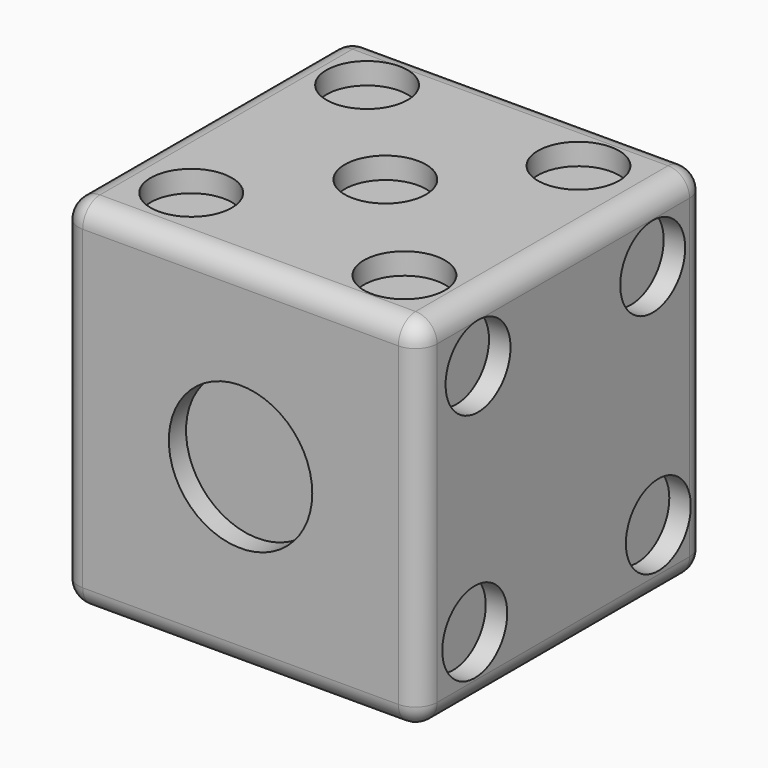
from build123d import *

# Parameters (mm, degrees)
F0_W          = 12.7
F0_H          = 12.7
F1_DEPTH      = 12.7
F2_R          = 2.54
F3_DEPTH      = 0.762
F4_R          = 1.4370558
F5_DEPTH      = 0.762
F6_R          = 1.4370558
F7_DEPTH      = 0.762
F8_R          = 1.4370558
F9_DEPTH      = 0.762
F10_R         = 1.4370558
F11_DEPTH     = 0.762
F12_T1_DEPTH  = 11.176
F12_T3_DEPTH  = 11.176
F12_T5_DEPTH  = 11.176
F12_S9_W      = 0.762
F12_S9_H      = 0.762
F12_T10_DEPTH = 0.762
F12_S15_W     = 0.762
F12_S15_H     = 0.762
F12_T16_DEPTH = 0.762
F12_S21_W     = 0.762
F12_S21_H     = 0.762
F12_T22_DEPTH = 0.762
F12_S27_W     = 0.762
F12_S27_H     = 0.762
F12_T28_DEPTH = 0.762
F12_S33_W     = 0.762
F12_S33_H     = 0.762
F12_T34_DEPTH = 0.762
F12_S39_W     = 0.762
F12_S39_H     = 0.762
F12_T40_DEPTH = 0.762
F12_S45_W     = 0.762
F12_S45_H     = 0.762
F12_T46_DEPTH = 0.762
F12_S51_W     = 0.762
F12_S51_H     = 0.762
F12_T52_DEPTH = 0.762
F13_R         = 1.4370558
F14_DEPTH     = 0.762


# Not quite as in the source:
# - a fillet or chamfer that OpenCascade refuses, or shapes differently, is made with other operations: its cross-section is extruded or revolved along the edge and cut away or added


with BuildPart() as f1:
    # F0 (on Front) → F1 (new body)
    with BuildSketch(Plane.XZ):
        Rectangle(F0_W, F0_H)
    extrude(amount=F1_DEPTH)

    # F2 (on face) → F3 (cut)
    with BuildSketch(Plane.XZ.offset(12.7)):
        Circle(F2_R)
    extrude(amount=-F3_DEPTH, mode=Mode.SUBTRACT)

    # F4 (on face) → F5 (cut)
    with BuildSketch(Plane(origin=(0, 0, 0), x_dir=(-1, 0, 0), z_dir=(0, 1, 0))):
        with Locations((-4.0605822578, 4.3273498304)):
            Circle(F4_R)
        with Locations((4.0411474183, -3.9733615704)):
            Circle(F4_R)
    extrude(amount=-F5_DEPTH, mode=Mode.SUBTRACT)

    # F6 (on face) → F7 (cut)
    with BuildSketch(Plane(origin=(-6.35, 0, 0), x_dir=(0, -1, 0), z_dir=(-1, 0, 0))):
        with Locations((6.2880520709, 0)):
            Circle(F6_R)
        with Locations((10.5908196419, -4.2169503868)):
            Circle(F6_R)
        with Locations((2.0048597362, 4.2917155661)):
            Circle(F6_R)
    extrude(amount=-F7_DEPTH, mode=Mode.SUBTRACT)

    # F8 (on face) → F9 (cut)
    with BuildSketch(Plane.YZ.offset(6.35)):
        with Locations((-10.1248482242, 4.1586253792)):
            Circle(F8_R)
        with Locations((-2.3929197341, 4.1189542972)):
            Circle(F8_R)
        with Locations((-10.2693093941, -4.0696617216)):
            Circle(F8_R)
        with Locations((-2.1438063122, -4.0340232663)):
            Circle(F8_R)
    extrude(amount=-F9_DEPTH, mode=Mode.SUBTRACT)

    # F10 (on face) → F11 (cut)
    with BuildSketch(Plane.XY.offset(6.35)):
        with Locations((0, -6.2898481265)):
            Circle(F10_R)
        with Locations((3.6543684546, -2.3101689294)):
            Circle(F10_R)
        with Locations((-3.9310273714, -2.1862694994)):
            Circle(F10_R)
        with Locations((-3.6943627056, -10.2638797835)):
            Circle(F10_R)
        with Locations((3.9920811541, -10.4369977489)):
            Circle(F10_R)
    extrude(amount=-F11_DEPTH, mode=Mode.SUBTRACT)

    # F12: fillet of radius 0.762 on 12 edges, made by hand

    # F12_s2 → F12_t1 (cut)
    with BuildSketch(Plane.YZ.offset(-5.588)):
        with BuildLine():
            ThreePointArc((-11.938, 6.35), (-12.4768153673, 6.1268153673), (-12.7, 5.588))
            Line((-12.7, 5.588), (-12.7, 6.35))
            Line((-12.7, 6.35), (-11.938, 6.35))
        make_face()
        with BuildLine():
            ThreePointArc((-0.762, 6.35), (-0.2231846327, 6.1268153673), (0, 5.588))
            Line((0, 5.588), (0, 6.35))
            Line((0, 6.35), (-0.762, 6.35))
        make_face()
        with BuildLine():
            ThreePointArc((-12.7, -5.588), (-12.4768153673, -6.1268153673), (-11.938, -6.35))
            Line((-11.938, -6.35), (-12.7, -6.35))
            Line((-12.7, -6.35), (-12.7, -5.588))
        make_face()
        with BuildLine():
            ThreePointArc((0, -5.588), (-0.2231846327, -6.1268153673), (-0.762, -6.35))
            Line((-0.762, -6.35), (0, -6.35))
            Line((0, -6.35), (0, -5.588))
        make_face()
    extrude(amount=F12_T1_DEPTH, mode=Mode.SUBTRACT)

    # F12_s4 → F12_t3 (cut)
    with BuildSketch(Plane.XZ.offset(0.762)):
        with BuildLine():
            ThreePointArc((-5.588, 6.35), (-6.1268153673, 6.1268153673), (-6.35, 5.588))
            Line((-6.35, 5.588), (-6.35, 6.35))
            Line((-6.35, 6.35), (-5.588, 6.35))
        make_face()
        with BuildLine():
            ThreePointArc((5.588, 6.35), (6.1268153673, 6.1268153673), (6.35, 5.588))
            Line((6.35, 5.588), (6.35, 6.35))
            Line((6.35, 6.35), (5.588, 6.35))
        make_face()
        with BuildLine():
            ThreePointArc((6.35, -5.588), (6.1268153673, -6.1268153673), (5.588, -6.35))
            Line((5.588, -6.35), (6.35, -6.35))
            Line((6.35, -6.35), (6.35, -5.588))
        make_face()
        with BuildLine():
            ThreePointArc((-6.35, -5.588), (-6.1268153673, -6.1268153673), (-5.588, -6.35))
            Line((-5.588, -6.35), (-6.35, -6.35))
            Line((-6.35, -6.35), (-6.35, -5.588))
        make_face()
    extrude(amount=F12_T3_DEPTH, mode=Mode.SUBTRACT)

    # F12_s6 → F12_t5 (cut)
    with BuildSketch(Plane.XY.offset(-5.588)):
        with BuildLine():
            ThreePointArc((6.35, -11.938), (6.1268153673, -12.4768153673), (5.588, -12.7))
            Line((5.588, -12.7), (6.35, -12.7))
            Line((6.35, -12.7), (6.35, -11.938))
        make_face()
        with BuildLine():
            ThreePointArc((-5.588, -12.7), (-6.1268153673, -12.4768153673), (-6.35, -11.938))
            Line((-6.35, -11.938), (-6.35, -12.7))
            Line((-6.35, -12.7), (-5.588, -12.7))
        make_face()
        with BuildLine():
            ThreePointArc((6.35, -0.762), (6.1268153673, -0.2231846327), (5.588, 0))
            Line((5.588, 0), (6.35, 0))
            Line((6.35, 0), (6.35, -0.762))
        make_face()
        with BuildLine():
            ThreePointArc((-5.588, 0), (-6.1268153673, -0.2231846327), (-6.35, -0.762))
            Line((-6.35, -0.762), (-6.35, 0))
            Line((-6.35, 0), (-5.588, 0))
        make_face()
    extrude(amount=F12_T5_DEPTH, mode=Mode.SUBTRACT)


with BuildPart() as f12_tool8:
    # F12_s9 → F12_t10 (new body)
    with BuildSketch(Plane.XY.offset(5.588)):
        with Locations((5.969, -12.319)):
            Rectangle(F12_S9_W, F12_S9_H)
    extrude(amount=F12_T10_DEPTH)

    # F12_s11 → F12_t12 (revolve, cut)
    with BuildSketch(Plane(origin=(5.588, -11.938, 5.588), x_dir=(-0.7071067812, 0.7071067812, 0), z_dir=(0.7071067812, 0.7071067812, 0))):
        with BuildLine():
            ThreePointArc((0, -0.762), (0.762, 0), (0, 0.762))
            Line((0, 0.762), (0, -0.762))
        make_face()
    revolve(axis=Axis((5.588, -11.938, 5.588), (0, 0, 1)), mode=Mode.SUBTRACT)


with BuildPart() as f1_1:
    add(f1.part)

    # F12_t7: cut F12_tool8
    add(f12_tool8.part, mode=Mode.SUBTRACT)


with BuildPart() as f12_tool14:
    # F12_s15 → F12_t16 (new body)
    with BuildSketch(Plane.XY.offset(5.588)):
        with Locations((-5.969, -12.319)):
            Rectangle(F12_S15_W, F12_S15_H)
    extrude(amount=F12_T16_DEPTH)

    # F12_s17 → F12_t18 (revolve, cut)
    with BuildSketch(Plane(origin=(-5.588, -11.938, 5.588), x_dir=(0.7071067812, 0.7071067812, 0), z_dir=(0.7071067812, -0.7071067812, 0))):
        with BuildLine():
            ThreePointArc((0, -0.762), (0.762, 0), (0, 0.762))
            Line((0, 0.762), (0, -0.762))
        make_face()
    revolve(axis=Axis((-5.588, -11.938, 5.588), (0, 0, 1)), mode=Mode.SUBTRACT)


with BuildPart() as f1_2:
    add(f1_1.part)

    # F12_t13: cut F12_tool14
    add(f12_tool14.part, mode=Mode.SUBTRACT)


with BuildPart() as f12_tool20:
    # F12_s21 → F12_t22 (new body)
    with BuildSketch(Plane.XY.offset(5.588)):
        with Locations((-5.969, -0.381)):
            Rectangle(F12_S21_W, F12_S21_H)
    extrude(amount=F12_T22_DEPTH)

    # F12_s23 → F12_t24 (revolve, cut)
    with BuildSketch(Plane(origin=(-5.588, -0.762, 5.588), x_dir=(0.7071067812, -0.7071067812, 0), z_dir=(-0.7071067812, -0.7071067812, 0))):
        with BuildLine():
            ThreePointArc((0, -0.762), (0.762, 0), (0, 0.762))
            Line((0, 0.762), (0, -0.762))
        make_face()
    revolve(axis=Axis((-5.588, -0.762, 5.588), (0, 0, 1)), mode=Mode.SUBTRACT)


with BuildPart() as f1_3:
    add(f1_2.part)

    # F12_t19: cut F12_tool20
    add(f12_tool20.part, mode=Mode.SUBTRACT)


with BuildPart() as f12_tool26:
    # F12_s27 → F12_t28 (new body)
    with BuildSketch(Plane.XY.offset(5.588)):
        with Locations((5.969, -0.381)):
            Rectangle(F12_S27_W, F12_S27_H)
    extrude(amount=F12_T28_DEPTH)

    # F12_s29 → F12_t30 (revolve, cut)
    with BuildSketch(Plane(origin=(5.588, -0.762, 5.588), x_dir=(-0.7071067812, -0.7071067812, 0), z_dir=(-0.7071067812, 0.7071067812, 0))):
        with BuildLine():
            ThreePointArc((0, -0.762), (0.762, 0), (0, 0.762))
            Line((0, 0.762), (0, -0.762))
        make_face()
    revolve(axis=Axis((5.588, -0.762, 5.588), (0, 0, 1)), mode=Mode.SUBTRACT)


with BuildPart() as f1_4:
    add(f1_3.part)

    # F12_t25: cut F12_tool26
    add(f12_tool26.part, mode=Mode.SUBTRACT)


with BuildPart() as f12_tool32:
    # F12_s33 → F12_t34 (new body)
    with BuildSketch(Plane.YZ.offset(5.588)):
        with Locations((-12.319, -5.969)):
            Rectangle(F12_S33_W, F12_S33_H)
    extrude(amount=F12_T34_DEPTH)

    # F12_s35 → F12_t36 (revolve, cut)
    with BuildSketch(Plane(origin=(5.588, -11.938, -5.588), x_dir=(0, 0.7071067812, 0.7071067812), z_dir=(0, 0.7071067812, -0.7071067812))):
        with BuildLine():
            ThreePointArc((0, -0.762), (0.762, 0), (0, 0.762))
            Line((0, 0.762), (0, -0.762))
        make_face()
    revolve(axis=Axis((5.588, -11.938, -5.588), (1, 0, 0)), mode=Mode.SUBTRACT)


with BuildPart() as f1_5:
    add(f1_4.part)

    # F12_t31: cut F12_tool32
    add(f12_tool32.part, mode=Mode.SUBTRACT)


with BuildPart() as f12_tool38:
    # F12_s39 → F12_t40 (new body)
    with BuildSketch(Plane.XY.offset(-5.588)):
        with Locations((-5.969, -12.319)):
            Rectangle(F12_S39_W, F12_S39_H)
    extrude(amount=-F12_T40_DEPTH)

    # F12_s41 → F12_t42 (revolve, cut)
    with BuildSketch(Plane(origin=(-5.588, -11.938, -5.588), x_dir=(0.7071067812, 0.7071067812, 0), z_dir=(-0.7071067812, 0.7071067812, 0))):
        with BuildLine():
            ThreePointArc((0, -0.762), (0.762, 0), (0, 0.762))
            Line((0, 0.762), (0, -0.762))
        make_face()
    revolve(axis=Axis((-5.588, -11.938, -5.588), (0, 0, -1)), mode=Mode.SUBTRACT)


with BuildPart() as f1_6:
    add(f1_5.part)

    # F12_t37: cut F12_tool38
    add(f12_tool38.part, mode=Mode.SUBTRACT)


with BuildPart() as f12_tool44:
    # F12_s45 → F12_t46 (new body)
    with BuildSketch(Plane.YZ.offset(5.588)):
        with Locations((-0.381, -5.969)):
            Rectangle(F12_S45_W, F12_S45_H)
    extrude(amount=F12_T46_DEPTH)

    # F12_s47 → F12_t48 (revolve, cut)
    with BuildSketch(Plane(origin=(5.588, -0.762, -5.588), x_dir=(0, -0.7071067812, 0.7071067812), z_dir=(0, 0.7071067812, 0.7071067812))):
        with BuildLine():
            ThreePointArc((0, -0.762), (0.762, 0), (0, 0.762))
            Line((0, 0.762), (0, -0.762))
        make_face()
    revolve(axis=Axis((5.588, -0.762, -5.588), (1, 0, 0)), mode=Mode.SUBTRACT)


with BuildPart() as f1_7:
    add(f1_6.part)

    # F12_t43: cut F12_tool44
    add(f12_tool44.part, mode=Mode.SUBTRACT)


with BuildPart() as f12_tool50:
    # F12_s51 → F12_t52 (new body)
    with BuildSketch(Plane.XZ.offset(0.762)):
        with Locations((-5.969, -5.969)):
            Rectangle(F12_S51_W, F12_S51_H)
    extrude(amount=-F12_T52_DEPTH)

    # F12_s53 → F12_t54 (revolve, cut)
    with BuildSketch(Plane(origin=(-5.588, -0.762, -5.588), x_dir=(0.7071067812, 0, 0.7071067812), z_dir=(-0.7071067812, 0, 0.7071067812))):
        with BuildLine():
            ThreePointArc((0, -0.762), (0.762, 0), (0, 0.762))
            Line((0, 0.762), (0, -0.762))
        make_face()
    revolve(axis=Axis((-5.588, -0.762, -5.588), (0, 1, 0)), mode=Mode.SUBTRACT)


with BuildPart() as f1_8:
    add(f1_7.part)

    # F12_t49: cut F12_tool50
    add(f12_tool50.part, mode=Mode.SUBTRACT)

    # F13 (on face) → F14 (cut)
    with BuildSketch(Plane(origin=(0, 0, -6.35), x_dir=(1, 0, 0), z_dir=(0, 0, -1))):
        with Locations((3.3344947733, 6.35)):
            Circle(F13_R)
        with Locations((3.3242953941, 9.9209658802)):
            Circle(F13_R)
        with Locations((3.3245715313, 2.7183145285)):
            Circle(F13_R)
        with Locations((-3.2171458006, 10.041509755)):
            Circle(F13_R)
        with Locations((-3.3451111522, 6.3969474286)):
            Circle(F13_R)
        with Locations((-3.2923812978, 2.8163562529)):
            Circle(F13_R)
    extrude(amount=-F14_DEPTH, mode=Mode.SUBTRACT)


solid = f1_8.part
